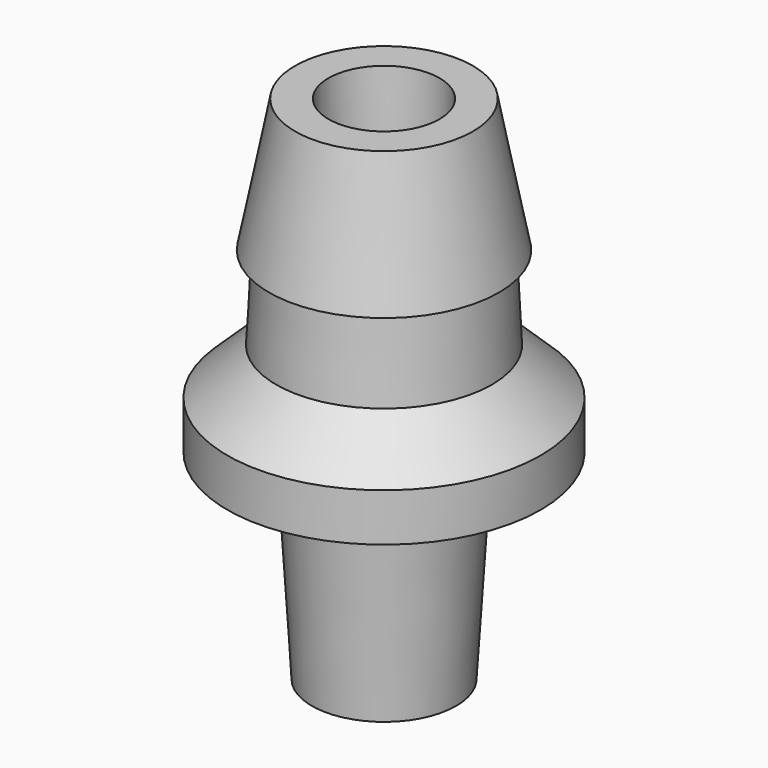
from build123d import *

# Parameters (mm, degrees)
F2_S5_R     = 3.5814
F2_T6_DEPTH = 7


# Not quite as in the source:
# - a fillet or chamfer that OpenCascade refuses, or shapes differently, is made with other operations: its cross-section is extruded or revolved along the edge and cut away or added


with BuildPart() as f1:
    # F0 (on Front) → F1 (revolve)
    with BuildSketch(Plane.XZ):
        Polygon((0.889, -4.572), (1.651, -4.572), (1.9304, 0), (3.5814, 0), (3.5814, 0.889), (2.5273, 0.889), (2.3749, 4.064), (2.6289, 4.064), (2.032, 7.112), (1.27, 7.112), align=None)
    revolve(axis=Axis((0, 0, 1.778), (0, 0, 1)))

    # F2: chamfer of 1.27 on 1 edges, made by hand


with BuildPart() as f2_tool2:
    # F2_s3 → F2_t4 (revolve)
    with BuildSketch(Plane.XZ):
        Polygon((3.7973, 0.889), (2.4664101048, 2.1575394833), (2.5273, 0.889), align=None)
    revolve(axis=Axis((0, 0, 0.889), (0, 0, 1)))

    # F2_s5 → F2_t6 (intersect, symmetric)
    with BuildSketch(Plane.XY.offset(1.5)):
        Circle(F2_S5_R)
    extrude(amount=F2_T6_DEPTH, both=True, mode=Mode.INTERSECT)


with BuildPart() as f1_1:
    add(f1.part)

    # F2_t1: union F2_tool2
    add(f2_tool2.part)


solid = f1_1.part
